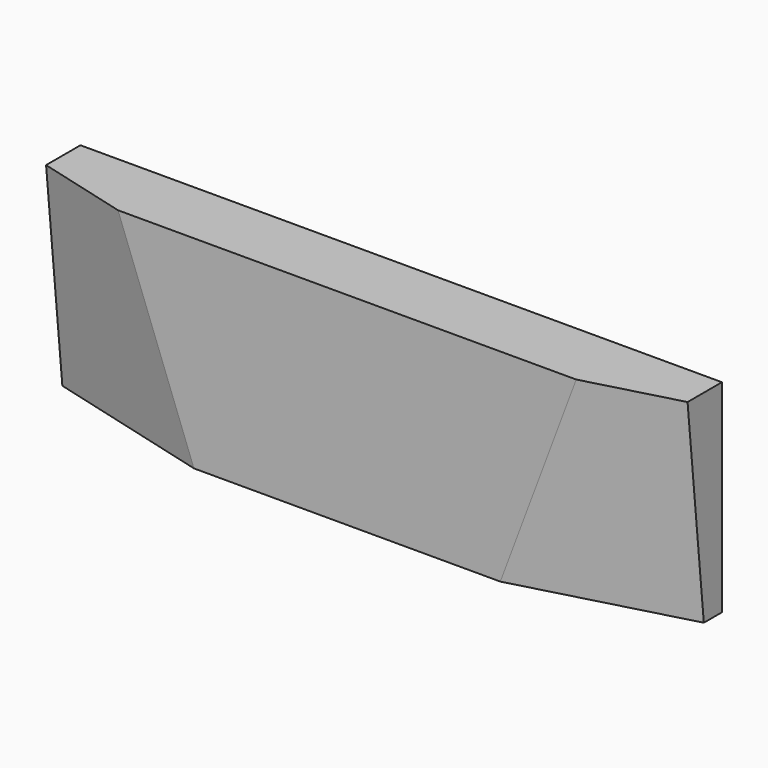
from build123d import *

# Parameters (mm, degrees)
F0_W     = 482.6
F0_H     = 50.8
F1_DEPTH = 152.4


# Not quite as in the source:
# - a pattern or mirror of a feature is missing from the dataset's text; its kind, count and spacing are read off the source's solid


with BuildPart() as f1:
    # F0 (on Top) → F1 (new body)
    with BuildSketch(Plane.XY):
        Rectangle(F0_W, F0_H)
    extrude(amount=F1_DEPTH)

    # F4: sweep along a path in F3
    with BuildLine(Plane(origin=(-241.3, 0, 0), x_dir=(0, -1, 0), z_dir=(-1, 0, 0))) as f4_path:
        Line((15.9376427472, 242.2395817821), (-8.382, 0))
    # F2 (on face) → F4 (sweep, cut)
    with BuildSketch(Plane(origin=(0, 0, 0), x_dir=(1, 0, 0), z_dir=(0, 0, -1))):
        Polygon((-241.3, 25.4), (-241.3, -8.382), (-115.2238596187, 25.4), align=None)
    f4 = sweep(path=f4_path.line, mode=Mode.SUBTRACT)

    # F4_copies: F4 across plane
    add(f4.mirror(Plane(origin=(0, 0, 0), x_dir=(0, 0, 1), z_dir=(1, 0, 0))), mode=Mode.SUBTRACT)


solid = f1.part
